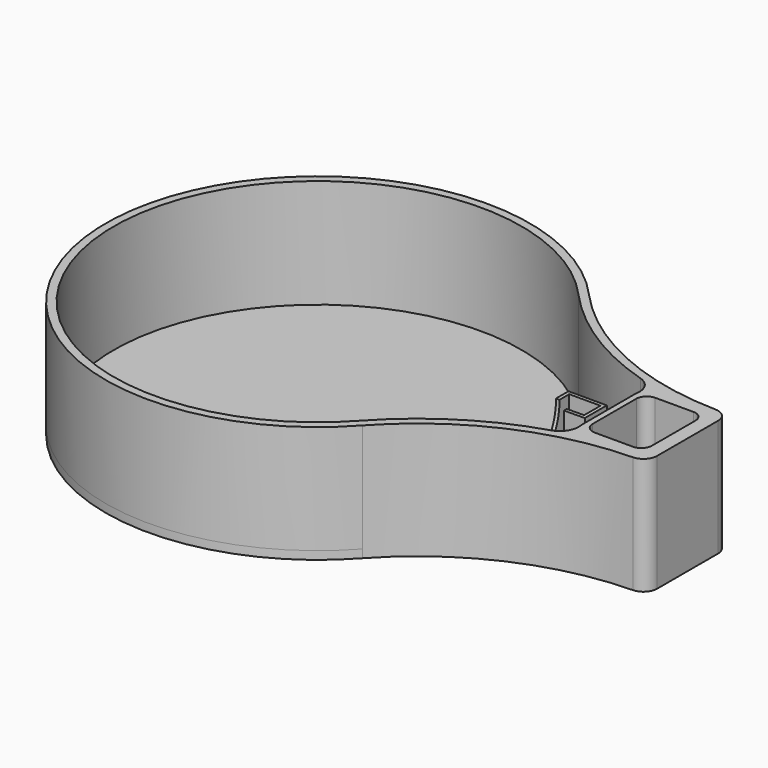
from build123d import *
from build123d import SkipClean  # not in build123d's __all__

# Parameters (mm, degrees)
F1_DEPTH  = 40
F2_DEPTH  = 3
F3_DEPTH  = 24
F4_DEPTH  = 40
F6_DEPTH  = 2.5
F7_W      = 6
F7_H      = 1.3
F8_DEPTH  = 13
F9_W      = 4
F9_H      = 2
F10_DEPTH = 6.5
F11_R     = 1.5
F12_DEPTH = 3.5
F13_R     = 5
F14_DEPTH = 2.5
F15_R     = 3.8627416998
F16_R     = 7
F17_R     = 7
F18_R     = 5


# Not quite as in the source:
# - after a boolean that leaves OpenCascade's solid faulty, fix() repairs it


with BuildPart() as f1:
    # F0 (on Top) → F1 (new body)
    with BuildSketch(Plane.XY):
        with BuildLine():
            ThreePointArc((136.0017471959, 19.0444356012), (93.4644134414, 27.0237675476), (58.1274125485, 52.0115819608))
            ThreePointArc((58.1274125485, 52.0115819608), (-1.3417961939, 78.0013424722), (-59.8907435455, 49.9999995776))
            ThreePointArc((-59.8907435455, 49.9999995776), (-77.9889397002, -0.003066533), (-59.8738076097, -49.9999995776))
            ThreePointArc((-59.8738076097, -49.9999995776), (-1.3426138919, -77.9810495035), (58.1087045089, -52.0122117666))
            ThreePointArc((58.1087045089, -52.0122117666), (93.4442134492, -27.0247840784), (135.9799137778, -19.0445627716))
            Line((135.9799137778, -19.0445627716), (136.0017471959, 19.0444356012))
        make_face()
        with BuildLine():
            ThreePointArc((55.9016994375, 50), (90.8688121766, 24.8773821457), (133, 16))
            Line((133, 16), (132.9816567922, -16.0002304621))
            ThreePointArc((132.9816567922, -16.0002304621), (90.8504689689, -24.8776126078), (55.8833562297, -50.0002304621))
            ThreePointArc((55.8833562297, -50.0002304621), (-75.0149890076, 0.0238973514), (55.9016994375, 50))
        make_face(mode=Mode.SUBTRACT)
    extrude(amount=F1_DEPTH)

    # F0 (on Top) → F2 (join)
    with BuildSketch(Plane.XY):
        with BuildLine():
            ThreePointArc((136.0017471959, 19.0444356012), (93.4644134414, 27.0237675476), (58.1274125485, 52.0115819608))
            ThreePointArc((58.1274125485, 52.0115819608), (-1.3417961939, 78.0013424722), (-59.8907435455, 49.9999995776))
            ThreePointArc((-59.8907435455, 49.9999995776), (-77.9889397002, -0.003066533), (-59.8738076097, -49.9999995776))
            ThreePointArc((-59.8738076097, -49.9999995776), (-1.3426138919, -77.9810495035), (58.1087045089, -52.0122117666))
            ThreePointArc((58.1087045089, -52.0122117666), (93.4442134492, -27.0247840784), (135.9799137778, -19.0445627716))
            Line((135.9799137778, -19.0445627716), (136.0017471959, 19.0444356012))
        make_face()
        with BuildLine():
            ThreePointArc((55.9016994375, 50), (90.8688121766, 24.8773821457), (133, 16))
            Line((133, 16), (132.9816567922, -16.0002304621))
            ThreePointArc((132.9816567922, -16.0002304621), (90.8504689689, -24.8776126078), (55.8833562297, -50.0002304621))
            ThreePointArc((55.8833562297, -50.0002304621), (-75.0149890076, 0.0238973514), (55.9016994375, 50))
        make_face(mode=Mode.SUBTRACT)
        with BuildLine():
            ThreePointArc((-59.8738076097, -49.9999995776), (-77.9889397002, -0.003066533), (-59.8907435455, 49.9999995776))
            ThreePointArc((-59.8907435455, 49.9999995776), (-78.014990719, -0.003070945), (-59.8738076097, -49.9999995776))
        make_face()
        with BuildLine():
            Line((106.9816567922, 16), (133, 16))
            ThreePointArc((133, 16), (90.8688121766, 24.8773821457), (55.9016994375, 50))
            ThreePointArc((55.9016994375, 50), (-75.0149890076, 0.0238973514), (55.8833562297, -50.0002304621))
            ThreePointArc((55.8833562297, -50.0002304621), (90.8504689689, -24.8776126078), (132.9816567922, -16.0002304621))
            Line((132.9816567922, -16.0002304621), (106.9816567922, -16.0002304621))
            Line((106.9816567922, -16.0002304621), (106.9816567922, 16))
        make_face()
        Polygon((71.8, 25.4997695379), (85.881656831, 25.4997695379), (85.881656831, 15.3997695379), (78.2822565953, 15.3042914831), (78.2659248228, 16.6041888918), (84.6000000387, 16.6837695379), (84.6000000387, 24.1997695379), (73.1, 24.1997695379), (73.1, -24.2002304621), (84.6000000387, -24.2002304621), (84.6000000387, -16.6047524073), (78.2822565953, -16.6047524073), (78.2822565953, -15.3047524073), (85.881656831, -15.4002304621), (85.881656831, -25.5002304621), (71.8, -25.5002304621), align=None, mode=Mode.SUBTRACT)
        Polygon((132.9816567922, -16.0002304621), (133, 16), (106.9816567922, 16), (106.9816567922, -16.0002304621), align=None)
        Polygon((109.1000003293, -13.881886925), (109.1000003293, 13.8816564629), (130.8804418356, 13.8816564629), (130.8645271863, -13.881886925), align=None, mode=Mode.SUBTRACT)
        Polygon((130.8804418356, 13.8816564629), (109.1000003293, 13.8816564629), (109.1000003293, -13.881886925), (130.8645271863, -13.881886925), align=None)
        Polygon((85.881656831, 15.3997695379), (85.881656831, 25.4997695379), (71.8, 25.4997695379), (71.8, -25.5002304621), (85.881656831, -25.5002304621), (85.881656831, -15.4002304621), (78.2822565953, -15.3047524073), (78.2822565953, -16.6047524073), (84.6000000387, -16.6047524073), (84.6000000387, -24.2002304621), (73.1, -24.2002304621), (73.1, 24.1997695379), (84.6000000387, 24.1997695379), (84.6000000387, 16.6837695379), (78.2659248228, 16.6041888918), (78.2822565953, 15.3042914831), align=None)
    with SkipClean():  # cleaning this boolean's faces spoils the solid; the shape is the same uncleaned
        extrude(amount=-F2_DEPTH)

    # F0 (on Top) → F3 (join)
    with BuildSketch(Plane.XY):
        Polygon((85.881656831, 15.3997695379), (85.881656831, 25.4997695379), (71.8, 25.4997695379), (71.8, -25.5002304621), (85.881656831, -25.5002304621), (85.881656831, -15.4002304621), (78.2822565953, -15.3047524073), (78.2822565953, -16.6047524073), (84.6000000387, -16.6047524073), (84.6000000387, -24.2002304621), (73.1, -24.2002304621), (73.1, 24.1997695379), (84.6000000387, 24.1997695379), (84.6000000387, 16.6837695379), (78.2659248228, 16.6041888918), (78.2822565953, 15.3042914831), align=None)
    extrude(amount=F3_DEPTH)

    add(f1.part.fix(), mode=Mode.REPLACE)

    # F0 (on Top) → F4 (join)
    with BuildSketch(Plane.XY):
        Polygon((132.9816567922, -16.0002304621), (133, 16), (106.9816567922, 16), (106.9816567922, -16.0002304621), align=None)
        Polygon((109.1000003293, -13.881886925), (109.1000003293, 13.8816564629), (130.8804418356, 13.8816564629), (130.8645271863, -13.881886925), align=None, mode=Mode.SUBTRACT)
    extrude(amount=F4_DEPTH)

    # F5 (on face) → F6 (cut)
    with BuildSketch(Plane(origin=(71.8, 0, 0), x_dir=(0, -1, 0), z_dir=(-1, 0, 0))):
        with BuildLine():
            Line((19.7002304621, 24), (-19.6997695379, 24))
            ThreePointArc((-19.6997695379, 24), (0.0002304621, 3.4999999987), (19.7002304621, 24))
        make_face()
    extrude(amount=-F6_DEPTH, mode=Mode.SUBTRACT)

    # F7 (on face) → F8 (join)
    with BuildSketch(Plane.XY):
        with Locations((97.1279456019, 6.8092534184)):
            Rectangle(F7_W, F7_H)
        with Locations((97.1279456019, -6.85)):
            Rectangle(F7_W, F7_H)
    extrude(amount=F8_DEPTH)

    # F9 (on face) → F10 (join)
    with BuildSketch(Plane.XY):
        with Locations((78.6196921468, 9)):
            Rectangle(F9_W, F9_H)
        with Locations((78.6196921468, -9)):
            Rectangle(F9_W, F9_H)
    extrude(amount=F10_DEPTH)

    # F11 (on face) → F12 (cut)
    with BuildSketch(Plane(origin=(106.9816567922, 0, 0), x_dir=(0, -1, 0), z_dir=(-1, 0, 0))):
        with Locations((0.0001152311, 28)):
            Circle(F11_R)
    extrude(amount=-F12_DEPTH, mode=Mode.SUBTRACT)

    # F13 (on face) → F14 (cut)
    with BuildSketch(Plane(origin=(106.9816567922, 0, 0), x_dir=(0, -1, 0), z_dir=(-1, 0, 0))):
        with Locations((0, 11.5517321974)):
            Circle(F13_R)
    extrude(amount=-F14_DEPTH, mode=Mode.SUBTRACT)

    # F15
    f15_edges = [f1.edges().sort_by_distance(p)[0] for p in [
        (130.880442, 13.881656, 20),
        (106.981657, 16, 20),
        (109.1, 13.881656, 20),
        (130.864527, -13.881887, 20),
        (106.981657, -16.00023, 20),
        (109.1, -13.881887, 20),
    ]]
    fillet(f15_edges, radius=F15_R)

    # F16
    f16_edges = [f1.edges().sort_by_distance(p)[0] for p in [
        (132.981657, -16.00023, 20),
    ]]
    fillet(f16_edges, radius=F16_R)

    # F17
    f17_edges = [f1.edges().sort_by_distance(p)[0] for p in [
        (133, 16, 20),
    ]]
    fillet(f17_edges, radius=F17_R)

    # F18
    f18_edges = [f1.edges().sort_by_distance(p)[0] for p in [
        (135.979914, -19.044563, 18.5),
        (136.001747, 19.044436, 18.5),
    ]]
    fillet(f18_edges, radius=F18_R)


solid = f1.part
